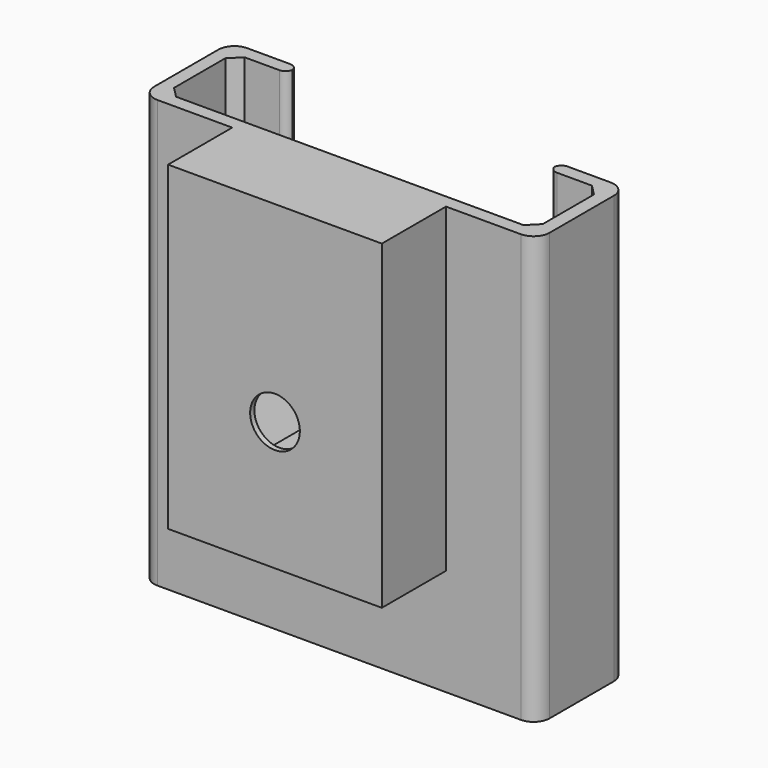
from build123d import *

# Parameters (mm, degrees)
F1_DEPTH      = 80
F0_W          = 2.5
F0_H          = 16
F0_W_2        = 6.5
F2_DEPTH      = 2.5
F3_SIZE       = 2
F4_R          = 3
F5_T1_DEPTH   = 87.5
F5_T3_DEPTH   = 16
F5_T8_DEPTH   = 16
F7_W          = 40
F7_H          = 60
F8_DEPTH      = 15
F6_R          = 4.65
F9_DEPTH      = 14
F9_DEPTH_BACK = 25
F10_R         = 4.65
F11_DEPTH     = 25


# Not quite as in the source:
# - a fillet or chamfer that OpenCascade refuses, or shapes differently, is made with other operations: its cross-section is extruded or revolved along the edge and cut away or added


with BuildPart() as f1:
    # F0 (on Top) → F1 (new body)
    with BuildSketch(Plane.XY):
        Polygon((-11.9039647728, 18.5), (-24.4039647728, 18.5), (-24.4039647728, -2.5), (49.5960352272, -2.5), (49.5960352272, 18.5), (37.0960352272, 18.5), (37.0960352272, 16), (44.5960352272, 16), (47.0960352272, 16), (47.0960352272, 0), (44.5960352272, 0), (-15.4039647728, 0), (-21.9039647728, 0), (-21.9039647728, 16), (-15.4039647728, 16), (-11.9039647728, 16), align=None)
    extrude(amount=F1_DEPTH)

    # F0 (on Top) → F2 (join)
    with BuildSketch(Plane.XY):
        with Locations((45.8460352272, 8)):
            Rectangle(F0_W, F0_H)
        with Locations((-18.6539647728, 8)):
            Rectangle(F0_W_2, F0_H)
    extrude(amount=F2_DEPTH)

    # F3
    f3_edges = [f1.edges().sort_by_distance(p)[0] for p in [
        (47.096035, 0, 41.25),
        (47.096035, 16, 41.25),
        (-21.903965, 0, 41.25),
        (-21.903965, 16, 41.25),
    ]]
    chamfer(f3_edges, length=F3_SIZE)

    # F4
    f4_edges = [f1.edges().sort_by_distance(p)[0] for p in [
        (-24.403965, 18.5, 40),
        (-24.403965, -2.5, 40),
        (49.596035, -2.5, 40),
        (49.596035, 18.5, 40),
    ]]
    fillet(f4_edges, radius=F4_R)

    # F5: fillet of radius 1.5 on 8 edges, made by hand

    # F5_s2 → F5_t1 (cut)
    with BuildSketch(Plane.XY.offset(-3.75)):
        with BuildLine():
            ThreePointArc((-11.9039647728, 17.5), (-12.343304601, 16.4393398282), (-13.4039647728, 16))
            Line((-13.4039647728, 16), (-11.9039647728, 16))
            Line((-11.9039647728, 16), (-11.9039647728, 17.5))
        make_face()
        with BuildLine():
            ThreePointArc((-13.4039647728, 18.5), (-12.343304601, 18.0606601718), (-11.9039647728, 17))
            Line((-11.9039647728, 17), (-11.9039647728, 18.5))
            Line((-11.9039647728, 18.5), (-13.4039647728, 18.5))
        make_face()
        with BuildLine():
            ThreePointArc((38.5960352272, 18.5), (37.5353750554, 18.0606601718), (37.0960352272, 17))
            Line((37.0960352272, 17), (37.0960352272, 18.5))
            Line((37.0960352272, 18.5), (38.5960352272, 18.5))
        make_face()
        with BuildLine():
            ThreePointArc((37.0960352272, 17.5), (37.5353750554, 16.4393398282), (38.5960352272, 16))
            Line((38.5960352272, 16), (37.0960352272, 16))
            Line((37.0960352272, 16), (37.0960352272, 17.5))
        make_face()
    extrude(amount=F5_T1_DEPTH, mode=Mode.SUBTRACT)

    # F5_s4 → F5_t3 (cut)
    with BuildSketch(Plane.XZ.offset(-16)):
        with BuildLine():
            ThreePointArc((46.0960352272, 0), (45.0353750554, 0.4393398282), (44.5960352272, 1.5))
            Line((44.5960352272, 1.5), (44.5960352272, 0))
            Line((44.5960352272, 0), (46.0960352272, 0))
        make_face()
        with BuildLine():
            ThreePointArc((-15.4039647728, 1), (-15.843304601, 2.0606601718), (-16.9039647728, 2.5))
            Line((-16.9039647728, 2.5), (-15.4039647728, 2.5))
            Line((-15.4039647728, 2.5), (-15.4039647728, 1))
        make_face()
        with BuildLine():
            ThreePointArc((-16.9039647728, 0), (-15.843304601, 0.4393398282), (-15.4039647728, 1.5))
            Line((-15.4039647728, 1.5), (-15.4039647728, 0))
            Line((-15.4039647728, 0), (-16.9039647728, 0))
        make_face()
    extrude(amount=F5_T3_DEPTH, mode=Mode.SUBTRACT)


with BuildPart() as f5_tool6:
    # F5_s7 → F5_t8 (new body)
    with BuildSketch(Plane.XZ.offset(-16)):
        with BuildLine():
            ThreePointArc((46.0960352272, 2.5), (45.0353750554, 2.0606601718), (44.5960352272, 1))
            Line((44.5960352272, 1), (44.5960352272, 2.5))
            Line((44.5960352272, 2.5), (46.0960352272, 2.5))
        make_face()
    extrude(amount=F5_T8_DEPTH)

    split(bisect_by=Plane(origin=(30.5480176136, 30.5480176136, 0), x_dir=(0, 0, 1), z_dir=(-0.7071067812, -0.7071067812, 0)), keep=Keep.TOP)

    split(bisect_by=Plane(origin=(22.5480176136, -22.5480176136, 0), x_dir=(0, 0, 1), z_dir=(-0.7071067812, 0.7071067812, 0)), keep=Keep.TOP)


with BuildPart() as f1_1:
    add(f1.part)

    # F5_t5: cut F5_tool6
    add(f5_tool6.part, mode=Mode.SUBTRACT)

    # F7 (on face) → F8 (join)
    with BuildSketch(Plane.XZ.offset(2.5)):
        with Locations((12.5960352272, 50)):
            Rectangle(F7_W, F7_H)
    extrude(amount=F8_DEPTH)

    # F6 (on face) → F9 (cut, two sides)
    with BuildSketch(Plane.XZ.offset(2.5)) as f9_sk:
        Polygon((20.8232765631, 44.1168472171), (16.7096558952, 51.2418472171), (8.4824145592, 51.2418472171), (4.3687938912, 44.1168472171), (8.4824145592, 36.9918472171), (16.7096558952, 36.9918472171), align=None)
        with Locations((12.5960352272, 44.1168472171)):
            Circle(F6_R, mode=Mode.SUBTRACT)
    extrude(amount=F9_DEPTH, mode=Mode.SUBTRACT)
    extrude(f9_sk.sketch, amount=-F9_DEPTH_BACK, mode=Mode.SUBTRACT)

    # F10 (on face) → F11 (cut)
    with BuildSketch(Plane(origin=(0, 0, 0), x_dir=(-1, 0, 0), z_dir=(0, 1, 0))):
        with Locations((-12.5960352272, 44.1168472171)):
            Circle(F10_R)
    extrude(amount=-F11_DEPTH, mode=Mode.SUBTRACT)


solid = f1_1.part
